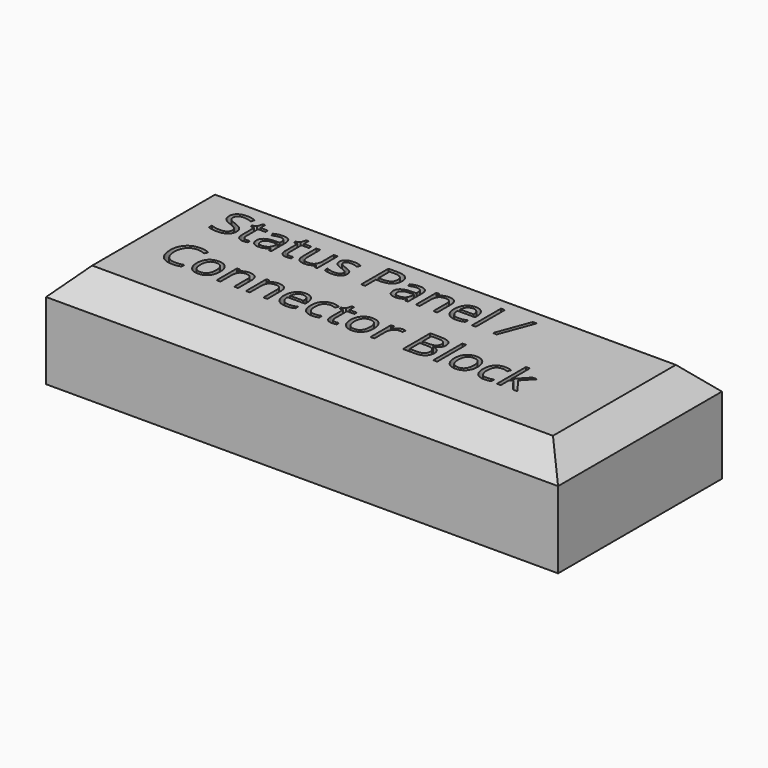
from build123d import *

# Parameters (mm, degrees)
F0_W         = 254
F0_H         = 101.6
F1_DEPTH     = 50.8
F2_TEXT_SIZE = 23.6881159556
F3_DEPTH     = 50.801
F4_SIZE      = 12.7


# Not quite as in the source:
# - Text() gives the source's letters only with a copy of the font that has no kerning and outlines rounded to 1/6400 em; it was checked with that copy


with BuildPart() as f1:
    # F0 (on Top) → F1 (new body)
    with BuildSketch(Plane.XY):
        with Locations((9.2491451651, -10.6424853611)):
            Rectangle(F0_W, F0_H)
    extrude(amount=F1_DEPTH)

    # F2 (on Top) → F3 (cut, through all)
    with BuildSketch(Plane.XY):
        with Locations((-91.0215855596, 4.0210136212)):
            Text('Status Panel /', F2_TEXT_SIZE, font='Open Sans', text_align=(TextAlign.LEFT, TextAlign.BOTTOM))
        with Locations((-91.0215855596, -28.1948240784)):
            Text('Connector Block', F2_TEXT_SIZE, font='Open Sans', text_align=(TextAlign.LEFT, TextAlign.BOTTOM))
    extrude(amount=F3_DEPTH, mode=Mode.SUBTRACT)

    # F4
    f4_edges = [f1.edges().sort_by_distance(p)[0] for p in [
        (9.249145, 40.157515, 50.8),
        (-117.750855, -10.642485, 50.8),
        (9.249145, -61.442485, 50.8),
        (136.249145, -10.642485, 50.8),
    ]]
    chamfer(f4_edges, length=F4_SIZE)


solid = f1.part
